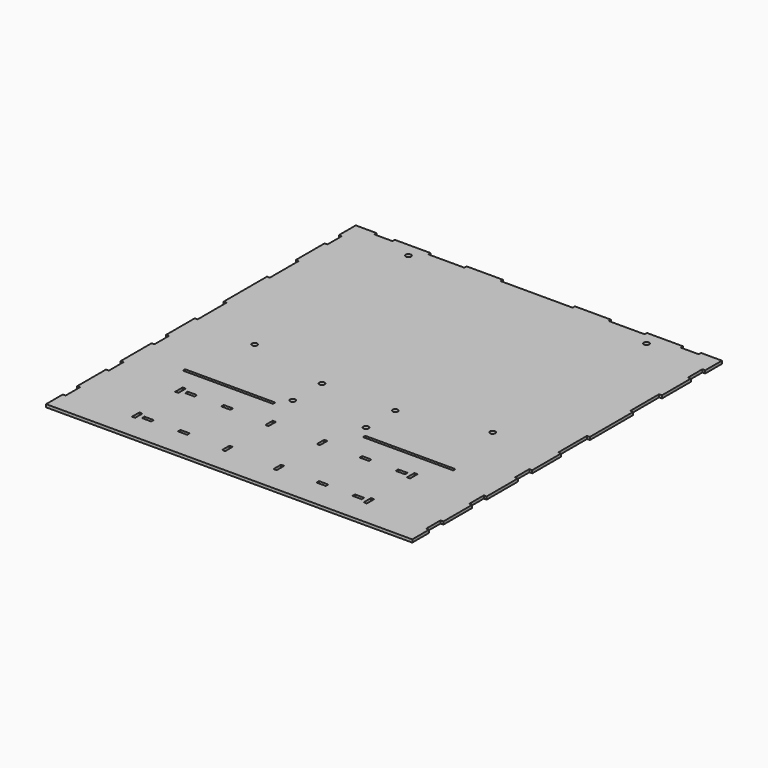
from build123d import *

# Parameters (mm, degrees)
F0_W     = 1.5875
F0_H     = 10
F0_H_2   = 20
F0_W_2   = 1.74625
F0_H_3   = 5.15
F0_W_3   = 5.15
F0_H_4   = 1.74625
F0_W_4   = 200
F0_H_5   = 1.5875
F0_W_5   = 50
F0_R     = 1.4732
F0_W_6   = 25
F0_H_6   = 30
F0_W_7   = 10
F0_W_8   = 20
F1_DEPTH = 1.5875


# Not quite as in the source:
# - a length typed as a fraction of an inch, garbled in the dataset ("3 / 203.2 mm" for 3/8 in), is restored


with BuildPart() as f1:
    # F0 (on Top) → F1 (new body)
    with BuildSketch(Plane.XY):
        with Locations((-100.79375, 176.5875)):
            Rectangle(F0_W, F0_H)
        with Locations((-100.79375, 36.5875)):
            Rectangle(F0_W, F0_H)
        with Locations((-100.79375, 61.5875)):
            Rectangle(F0_W, F0_H_2)
        with Locations((100.79375, 176.5875)):
            Rectangle(F0_W, F0_H)
        with Locations((100.79375, 36.5875)):
            Rectangle(F0_W, F0_H)
        with Locations((100.79375, 61.5875)):
            Rectangle(F0_W, F0_H_2)
        Polygon((100, 10), (100, 20), (-100, 20), (-100, 10), (-100, -10), (-100, -20), (100, -20), (100, -10), align=None)
        with Locations((-64.2875, -15)):
            Rectangle(F0_W_2, F0_H_3, mode=Mode.SUBTRACT)
        with Locations((-58.414375, -15)):
            Rectangle(F0_W_3, F0_H_4, mode=Mode.SUBTRACT)
        with Locations((-64.2875, 15)):
            Rectangle(F0_W_2, F0_H_3, mode=Mode.SUBTRACT)
        with Locations((-58.414375, 15)):
            Rectangle(F0_W_3, F0_H_4, mode=Mode.SUBTRACT)
        with Locations((-38.414375, -15)):
            Rectangle(F0_W_3, F0_H_4, mode=Mode.SUBTRACT)
        with Locations((-14.2875, -15)):
            Rectangle(F0_W_2, F0_H_3, mode=Mode.SUBTRACT)
        with Locations((-38.414375, 15)):
            Rectangle(F0_W_3, F0_H_4, mode=Mode.SUBTRACT)
        with Locations((-14.2875, 15)):
            Rectangle(F0_W_2, F0_H_3, mode=Mode.SUBTRACT)
        with Locations((14.2875, -15)):
            Rectangle(F0_W_2, F0_H_3, mode=Mode.SUBTRACT)
        with Locations((38.414375, -15)):
            Rectangle(F0_W_3, F0_H_4, mode=Mode.SUBTRACT)
        with Locations((14.2875, 15)):
            Rectangle(F0_W_2, F0_H_3, mode=Mode.SUBTRACT)
        with Locations((38.414375, 15)):
            Rectangle(F0_W_3, F0_H_4, mode=Mode.SUBTRACT)
        with Locations((58.414375, -15)):
            Rectangle(F0_W_3, F0_H_4, mode=Mode.SUBTRACT)
        with Locations((64.2875, -15)):
            Rectangle(F0_W_2, F0_H_3, mode=Mode.SUBTRACT)
        with Locations((58.414375, 15)):
            Rectangle(F0_W_3, F0_H_4, mode=Mode.SUBTRACT)
        with Locations((64.2875, 15)):
            Rectangle(F0_W_2, F0_H_3, mode=Mode.SUBTRACT)
        Polygon((-100, 20), (100, 20), (100, 30), (75, 30), (25, 30), (-25, 30), (-75, 30), (-100, 30), align=None)
        with Locations((0, -25)):
            Rectangle(F0_W_4, F0_H)
        with Locations((-100.79375, 0)):
            Rectangle(F0_W, F0_H_2)
        with Locations((100.79375, 0)):
            Rectangle(F0_W, F0_H_2)
        with Locations((100.79375, 25)):
            Rectangle(F0_W, F0_H)
        with Locations((100.79375, -25)):
            Rectangle(F0_W, F0_H)
        with Locations((-100.79375, 25)):
            Rectangle(F0_W, F0_H)
        with Locations((-100.79375, -25)):
            Rectangle(F0_W, F0_H)
        Polygon((101.5875, -30), (100, -30), (-100, -30), (-100, -31.5875), (101.5875, -31.5875), align=None)
        with Locations((-100.79375, 30.79375)):
            Rectangle(F0_W, F0_H_5)
        with Locations((0, 30.79375)):
            Rectangle(F0_W_5, F0_H_5)
        with Locations((100.79375, 30.79375)):
            Rectangle(F0_W, F0_H_5)
        with Locations((-100.79375, -30.79375)):
            Rectangle(F0_W, F0_H_5)
        Polygon((75, 31.5875), (100, 31.5875), (100, 41.5875), (100, 51.5875), (100, 71.5875), (100, 91.5875), (100, 121.5875), (100, 141.5875), (100, 161.5875), (100, 171.5875), (100, 181.5875), (90, 181.5875), (80, 181.5875), (60, 181.5875), (40, 181.5875), (20, 181.5875), (-20, 181.5875), (-40, 181.5875), (-60, 181.5875), (-80, 181.5875), (-90, 181.5875), (-100, 181.5875), (-100, 171.5875), (-100, 161.5875), (-100, 141.5875), (-100, 121.5875), (-100, 91.5875), (-100, 71.5875), (-100, 51.5875), (-100, 41.5875), (-100, 31.5875), (-75, 31.5875), (-25, 31.5875), (25, 31.5875), align=None)
        with Locations((-66.04, 68.5975)):
            Circle(F0_R, mode=Mode.SUBTRACT)
        with Locations((-20.32, 37.8975)):
            Circle(F0_R, mode=Mode.SUBTRACT)
        with Locations((-20.32, 58.2175)):
            Circle(F0_R, mode=Mode.SUBTRACT)
        with Locations((20.32, 37.8975)):
            Circle(F0_R, mode=Mode.SUBTRACT)
        with Locations((20.32, 58.2175)):
            Circle(F0_R, mode=Mode.SUBTRACT)
        with Locations((66.04, 68.5975)):
            Circle(F0_R, mode=Mode.SUBTRACT)
        with Locations((-66.04, 175.2775)):
            Circle(F0_R, mode=Mode.SUBTRACT)
        with Locations((66.04, 175.2775)):
            Circle(F0_R, mode=Mode.SUBTRACT)
        with Locations((87.5, 30.79375)):
            Rectangle(F0_W_6, F0_H_5)
        with Locations((-87.5, 30.79375)):
            Rectangle(F0_W_6, F0_H_5)
        with Locations((-100.79375, 106.5875)):
            Rectangle(F0_W, F0_H_6)
        with Locations((-100.79375, 151.5875)):
            Rectangle(F0_W, F0_H_2)
        with Locations((100.79375, 151.5875)):
            Rectangle(F0_W, F0_H_2)
        with Locations((100.79375, 106.5875)):
            Rectangle(F0_W, F0_H_6)
        with Locations((95, 182.38125)):
            Rectangle(F0_W_7, F0_H_5)
        with Locations((100.79375, 182.38125)):
            Rectangle(F0_W, F0_H_5)
        with Locations((-100.79375, 182.38125)):
            Rectangle(F0_W, F0_H_5)
        with Locations((-95, 182.38125)):
            Rectangle(F0_W_7, F0_H_5)
        with Locations((-70, 182.38125)):
            Rectangle(F0_W_8, F0_H_5)
        with Locations((-30, 182.38125)):
            Rectangle(F0_W_8, F0_H_5)
        with Locations((70, 182.38125)):
            Rectangle(F0_W_8, F0_H_5)
        with Locations((30, 182.38125)):
            Rectangle(F0_W_8, F0_H_5)
    extrude(amount=F1_DEPTH)


solid = f1.part
